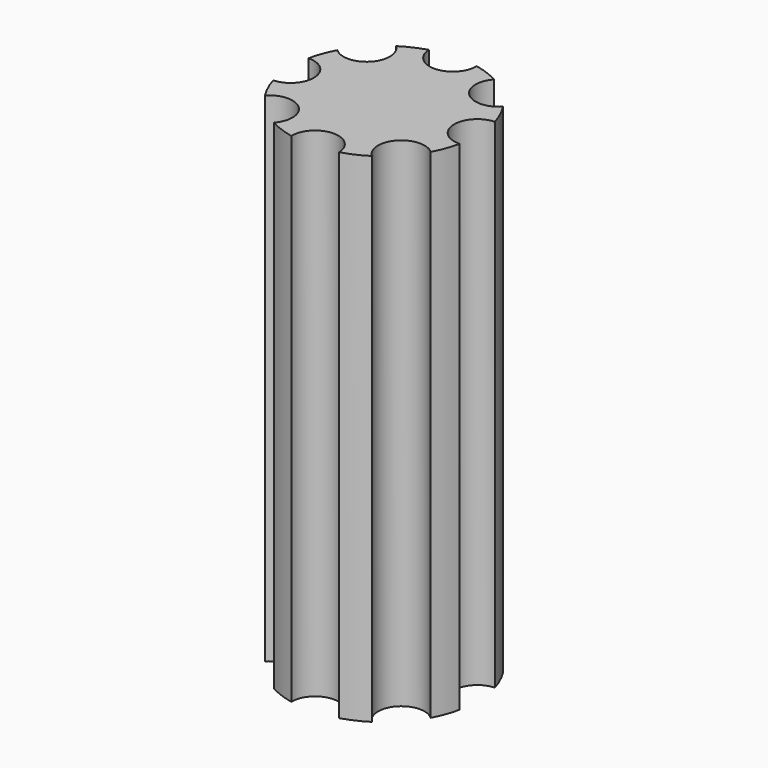
from build123d import *

# Parameters (mm, degrees)
F1_DEPTH = 40


with BuildPart() as f1:
    # F0 (on Top) → F1 (new body)
    with BuildSketch(Plane.XY):
        with BuildLine():
            ThreePointArc((7.3323928732, -1.5767101044), (5.4077667076, 0.2125573054), (7.1860144522, 2.1473696218))
            ThreePointArc((7.1860144522, 2.1473696218), (6.8110241928, 3.1400556437), (6.2996871297, 4.0698823162))
            ThreePointArc((6.2996871297, 4.0698823162), (3.673567798, 3.974169222), (3.5628599276, 6.5996991701))
            ThreePointArc((3.5628599276, 6.5996991701), (2.5957667546, 7.0364760325), (1.5767101044, 7.3323928732))
            ThreePointArc((1.5767101044, 7.3323928732), (-0.2125573054, 5.4077667076), (-2.1473696218, 7.1860144522))
            ThreePointArc((-2.1473696218, 7.1860144522), (-3.1400556437, 6.8110241928), (-4.0698823162, 6.2996871297))
            ThreePointArc((-4.0698823162, 6.2996871297), (-3.974169222, 3.673567798), (-6.5996991701, 3.5628599276))
            ThreePointArc((-6.5996991701, 3.5628599276), (-7.0364760325, 2.5957667546), (-7.3323928732, 1.5767101044))
            ThreePointArc((-7.3323928732, 1.5767101044), (-5.4077667076, -0.2125573054), (-7.1860144522, -2.1473696218))
            ThreePointArc((-7.1860144522, -2.1473696218), (-6.8110241928, -3.1400556437), (-6.2996871297, -4.0698823162))
            ThreePointArc((-6.2996871297, -4.0698823162), (-3.673567798, -3.974169222), (-3.5628599276, -6.5996991701))
            ThreePointArc((-3.5628599276, -6.5996991701), (-2.5957667546, -7.0364760325), (-1.5767101044, -7.3323928732))
            ThreePointArc((-1.5767101044, -7.3323928732), (0.2125573054, -5.4077667076), (2.1473696218, -7.1860144522))
            ThreePointArc((2.1473696218, -7.1860144522), (3.1400556437, -6.8110241928), (4.0698823162, -6.2996871297))
            ThreePointArc((4.0698823162, -6.2996871297), (3.974169222, -3.673567798), (6.5996991701, -3.5628599276))
            ThreePointArc((6.5996991701, -3.5628599276), (7.0364760325, -2.5957667546), (7.3323928732, -1.5767101044))
        make_face()
    extrude(amount=F1_DEPTH)


solid = f1.part
